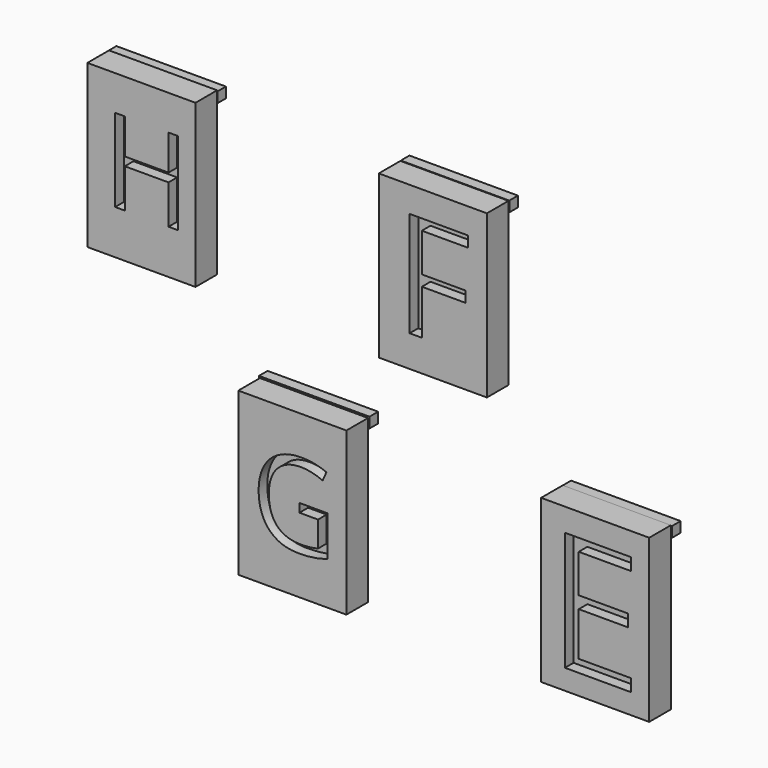
from build123d import *

# Parameters (mm, degrees)
F0_W           = 25.4
F0_H           = 38.1
F1_DEPTH       = 6.35
F2_R           = 3.81
F3_DEPTH       = 2.54
F5_TEXT_SIZE   = 39.1357293766
F5_TEXT_SIZE_2 = 34.5850544464
F5_TEXT_SIZE_3 = 27.3039978411
F6_DEPTH       = 25.4
F7_W           = 25.730624795
F7_H           = 2.4505369365
F8_DEPTH       = 2.54
F7_W_2         = 25.4855751991
F7_W_3         = 25.7306285203
F7_W_4         = 25.9756827727
F7_H_2         = 2.4505350739


# Not quite as in the source:
# - Text() gives the source's letters only with a copy of the font that has no kerning and outlines rounded to 1/6400 em; it was checked with that copy


with BuildPart() as f1:
    # F0 (on Front) → F1 (new body)
    with BuildSketch(Plane.XZ):
        with Locations((-46.0602159804, 19.2970331914)):
            Rectangle(F0_W, F0_H)
    extrude(amount=F1_DEPTH)

    # F2 (on Front) → F3, piece 2 (join)
    with BuildSketch(Plane.XZ):
        with Locations((-40.9802159804, 28.1870331914)):
            Circle(F2_R)
        with Locations((-51.1402159804, 18.0270331914)):
            Circle(F2_R)
        with Locations((-40.9802159804, 18.0270331914)):
            Circle(F2_R)
    extrude(amount=-F3_DEPTH)


with BuildPart() as f1b:
    # F0 (on Front) → F1, piece 2 (new body)
    with BuildSketch(Plane.XZ):
        with Locations((-10.603061258, -36.9614025138)):
            Rectangle(F0_W, F0_H)
    extrude(amount=F1_DEPTH)

    # F2 (on Front) → F3, piece 4 (join)
    with BuildSketch(Plane.XZ):
        with Locations((-5.523061258, -38.2314025138)):
            Circle(F2_R)
        with Locations((-15.683061258, -28.0714025138)):
            Circle(F2_R)
        with Locations((-5.523061258, -28.0714025138)):
            Circle(F2_R)
        with Locations((-15.683061258, -38.2314025138)):
            Circle(F2_R)
    extrude(amount=-F3_DEPTH)


with BuildPart() as f1c:
    # F0 (on Front) → F1, piece 3 (new body)
    with BuildSketch(Plane.XZ):
        with Locations((60.5514380593, -36.0065931796)):
            Rectangle(F0_W, F0_H)
    extrude(amount=F1_DEPTH)

    # F2 (on Front) → F3, piece 3 (join)
    with BuildSketch(Plane.XZ):
        with Locations((65.6314380593, -27.1165931796)):
            Circle(F2_R)
        with Locations((55.4714380593, -37.2765931796)):
            Circle(F2_R)
    extrude(amount=-F3_DEPTH)


with BuildPart() as f1d:
    # F0 (on Front) → F1, piece 4 (new body)
    with BuildSketch(Plane.XZ):
        with Locations((22.4085926682, 18.6961098781)):
            Rectangle(F0_W, F0_H)
    extrude(amount=F1_DEPTH)

    # F2 (on Front) → F3 (join)
    with BuildSketch(Plane.XZ):
        with Locations((27.4885926682, 17.4261098781)):
            Circle(F2_R)
        with Locations((27.4885926682, 27.5861098781)):
            Circle(F2_R)
        with Locations((17.3285926682, 27.5861098781)):
            Circle(F2_R)
    extrude(amount=-F3_DEPTH)


with BuildPart() as f6_tool:
    # F5 (on offset) → F6 (new body)
    with BuildSketch(Plane.XZ.offset(3.81)):
        with Locations((49.6037527919, -50.2979531884)):
            Text('E', F5_TEXT_SIZE, font='Open Sans', text_align=(TextAlign.LEFT, TextAlign.BOTTOM))
        with Locations((13.5624781251, 7.0404391736)):
            Text('F', F5_TEXT_SIZE_2, font='Open Sans', text_align=(TextAlign.LEFT, TextAlign.BOTTOM))
        with Locations((-20.1852573082, -46.6938279569)):
            Text('G', F5_TEXT_SIZE_3, font='Open Sans', text_align=(TextAlign.LEFT, TextAlign.BOTTOM))
        with Locations((-54.9159273505, 10.6445644051)):
            Text('H', F5_TEXT_SIZE_3, font='Open Sans', text_align=(TextAlign.LEFT, TextAlign.BOTTOM))
    extrude(amount=F6_DEPTH)


with BuildPart() as f1_1:
    add(f1.part)

    # F6: cut by f6_tool
    add(f6_tool.part, mode=Mode.SUBTRACT)

    # F7 (on Front) → F8, piece 3 (join)
    with BuildSketch(Plane.XZ):
        with Locations((-46.1926031858, 36.8805658072)):
            Rectangle(F7_W_3, F7_H)
    extrude(amount=-F8_DEPTH)


with BuildPart() as f1b_1:
    add(f1b.part)

    # F6: cut by f6_tool
    add(f6_tool.part, mode=Mode.SUBTRACT)

    # F7 (on Front) → F8, piece 4 (join)
    with BuildSketch(Plane.XZ):
        with Locations((-10.5373053811, -18.7466004863)):
            Rectangle(F7_W_4, F7_H_2)
    extrude(amount=-F8_DEPTH)


with BuildPart() as f1c_1:
    add(f1c.part)

    # F6: cut by f6_tool
    add(f6_tool.part, mode=Mode.SUBTRACT)

    # F7 (on Front) → F8 (join)
    with BuildSketch(Plane.XZ):
        with Locations((60.6507658958, -18.2564929128)):
            Rectangle(F7_W, F7_H)
    extrude(amount=-F8_DEPTH)


with BuildPart() as f1d_1:
    add(f1d.part)

    # F6: cut by f6_tool
    add(f6_tool.part, mode=Mode.SUBTRACT)

    # F7 (on Front) → F8, piece 2 (join)
    with BuildSketch(Plane.XZ):
        with Locations((22.5449316204, 36.6355124861)):
            Rectangle(F7_W_2, F7_H)
    extrude(amount=-F8_DEPTH)


solid = Compound([f1_1.part, f1b_1.part, f1c_1.part, f1d_1.part])
